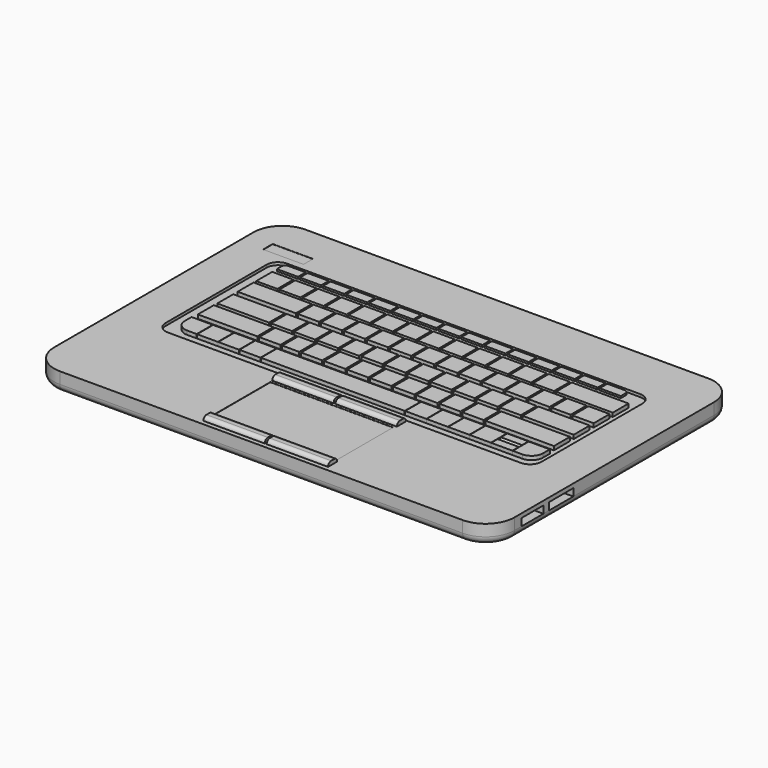
from build123d import *

# Parameters (mm, degrees)
F1_DEPTH  = 12.7
F2_R      = 5.08
F4_DEPTH  = 1.778
F5_W      = 13.7414
F5_H      = 13.2334
F5_W_2    = 13.9954
F5_W_3    = 95.25
F5_H_2    = 13.2237430662
F5_H_3    = 6.6167
F6_DEPTH  = 2.54
F7_SIZE   = 1.27
F8_SIZE   = 1.27
F9_W      = 13.9954
F9_H      = 13.2334
F9_W_2    = 12.7297410883
F9_W_3    = 11.1980646137
F9_W_4    = 13.97
F9_W_5    = 39.3358543515
F9_W_6    = 45.363843441
F9_W_7    = 34.2387035489
F9_W_8    = 33.7878703395
F9_W_9    = 38.5862437279
F9_W_10   = 37.5577136874
F9_H_2    = 13.1128338855
F10_DEPTH = 2.54
F11_W     = 40.64
F11_H     = 7.62
F12_DEPTH = 2.54
F13_R     = 2.53999
F14_R     = 2.53999
F15_R     = 2.53999
F16_W     = 81.28
F16_H     = 46.99
F17_DEPTH = 0.127
F19_DEPTH = 1.27
F18_W     = 13.9954
F18_H     = 6.3754
F20_W     = 26.701785624
F20_H     = 7.8833848238
F21_DEPTH = 0.127
F22_W     = 18.1714147329
F22_H     = 4.8768
F22_W_2   = 19.9380852282
F22_H_2   = 4.8890416828
F23_DEPTH = 12.7


# Not quite as in the source:
# - a fillet or chamfer is up to 0.001 mm smaller than in the source, because OpenCascade refuses the exact size


with BuildPart() as f1:
    # F0 (on Top) → F1 (new body)
    with BuildSketch(Plane.XY):
        with BuildLine():
            Line((133.35, 101.6), (-133.35, 101.6))
            ThreePointArc((-133.35, 101.6), (-146.8203841816, 96.0203841816), (-152.4, 82.55))
            Line((-152.4, 82.55), (-152.4, -82.55))
            ThreePointArc((-152.4, -82.55), (-146.8203841816, -96.0203841816), (-133.35, -101.6))
            Line((-133.35, -101.6), (133.35, -101.6))
            ThreePointArc((133.35, -101.6), (146.8203841816, -96.0203841816), (152.4, -82.55))
            Line((152.4, -82.55), (152.4, 82.55))
            ThreePointArc((152.4, 82.55), (146.8203841816, 96.0203841816), (133.35, 101.6))
        make_face()
    extrude(amount=F1_DEPTH)

    # F2
    f2_edges = [f1.edges().sort_by_distance(p)[0] for p in [
        (0, -101.6, 0),
    ]]
    fillet(f2_edges, radius=F2_R)

    # F3 (on face) → F4 (cut)
    with BuildSketch(Plane.XY.offset(12.7)):
        with BuildLine():
            ThreePointArc((-124.46, -25.1829952943), (-122.2281536726, -30.571148967), (-116.84, -32.8029952943))
            Line((-116.84, -32.8029952943), (116.84, -32.8029952943))
            ThreePointArc((116.84, -32.8029952943), (122.2281536726, -30.571148967), (124.46, -25.1829952943))
            Line((124.46, -25.1829952943), (124.46, 58.3147651076))
            ThreePointArc((124.46, 58.3147651076), (122.2281536726, 63.7029187803), (116.84, 65.9347651076))
            Line((116.84, 65.9347651076), (-116.84, 65.9347651076))
            ThreePointArc((-116.84, 65.9347651076), (-122.2281536726, 63.7029187803), (-124.46, 58.3147651076))
            Line((-124.46, 58.3147651076), (-124.46, -25.1829952943))
        make_face()
    extrude(amount=-F4_DEPTH, mode=Mode.SUBTRACT)

    # F5 (on face) → F6 (join, symmetric)
    with BuildSketch(Plane.XY.offset(10.922)):
        with BuildLine():
            Line((-103.2148086897, -12.7556547022), (-117.2102086897, -12.7556547022))
            Line((-117.2102086897, -12.7556547022), (-117.2102086897, -18.3690547022))
            ThreePointArc((-117.2102086897, -18.3690547022), (-114.9783623623, -23.7572083749), (-109.5902086897, -25.9890547022))
            Line((-109.5902086897, -25.9890547022), (-103.2148086897, -25.9890547022))
            Line((-103.2148086897, -25.9890547022), (-103.2148086897, -12.7556547022))
        make_face()
        with Locations((-96.0901086897, -19.3723547022)):
            Rectangle(F5_W, F5_H)
        with Locations((-82.0947086897, -19.3723547022)):
            Rectangle(F5_W, F5_H)
        with Locations((-67.9723086897, -19.3723547022)):
            Rectangle(F5_W_2, F5_H)
        with Locations((-13.0956086897, -19.3771831691)):
            Rectangle(F5_W_3, F5_H_2)
        with Locations((41.7810913103, -19.3723547022)):
            Rectangle(F5_W_2, F5_H)
        with Locations((56.0304913103, -19.3723547022)):
            Rectangle(F5_W_2, F5_H)
        with Locations((70.2798913103, -19.3723547022)):
            Rectangle(F5_W_2, F5_H)
        Polygon((91.2729913103, -12.7556547022), (77.5315913103, -12.7556547022), (77.5315913103, -25.9890547022), (91.5269913103, -25.9890547022), (91.5269913103, -12.7556547022), align=None)
        with BuildLine():
            Line((120.0257913103, -12.7556547022), (106.0303913103, -12.7556547022))
            Line((106.0303913103, -12.7556547022), (106.0303913103, -25.9890547022))
            Line((106.0303913103, -25.9890547022), (112.4057913103, -25.9890547022))
            ThreePointArc((112.4057913103, -25.9890547022), (117.793944983, -23.7572083749), (120.0257913103, -18.3690547022))
            Line((120.0257913103, -18.3690547022), (120.0257913103, -12.7556547022))
        make_face()
        Polygon((105.7763913103, -19.1183547022), (105.7763913103, -12.6286547022), (91.7809913103, -12.6286547022), (91.7809913103, -19.2453547022), (105.7763913103, -19.2453547022), align=None)
        with Locations((98.7786913103, -22.6807047022)):
            Rectangle(F5_W_2, F5_H_3)
    extrude(amount=F6_DEPTH, both=True)

    # F7
    f7_edges = [f1.edges().sort_by_distance(p)[0] for p in [
        (98.778691, -19.245355, 13.462),
    ]]
    chamfer(f7_edges, length=F7_SIZE)

    # F8
    f8_edges = [f1.edges().sort_by_distance(p)[0] for p in [
        (98.778691, -19.372355, 13.462),
    ]]
    chamfer(f8_edges, length=F8_SIZE)

    # F9 (on face) → F10 (join)
    with BuildSketch(Plane.XY.offset(10.922)):
        with Locations((-69.4690281525, 30.8539665655)):
            Rectangle(F9_W, F9_H)
        with Locations((-54.2036281525, 30.8539665655)):
            Rectangle(F9_W, F9_H)
        Polygon((-31.9405281525, 24.2372665655), (-31.9405281525, 37.4706665655), (-34.4356895394, 37.4706665655), (-45.9359281525, 37.4706665655), (-45.9359281525, 24.2372665655), align=None)
        Polygon((-16.6751281525, 37.4187609684), (-30.6705281525, 37.4814295383), (-30.6705281525, 24.2480295383), (-16.6751281525, 24.2480295383), align=None)
        with Locations((22.1233718475, 30.8539665655)):
            Rectangle(F9_W, F9_H)
        with Locations((37.3887718475, 30.8539665655)):
            Rectangle(F9_W, F9_H)
        with Locations((6.8579718475, 30.8539665655)):
            Rectangle(F9_W, F9_H)
        with Locations((-8.4074281525, 30.8539665655)):
            Rectangle(F9_W, F9_H)
        with Locations((52.6541718475, 30.8539665655)):
            Rectangle(F9_W, F9_H)
        with Locations((67.9195718475, 30.8539665655)):
            Rectangle(F9_W, F9_H)
        with Locations((97.8175423916, 30.8539665655)):
            Rectangle(F9_W_2, F9_H)
        with Locations((83.1849718475, 30.8539665655)):
            Rectangle(F9_W, F9_H)
        with Locations((-41.1575174346, -1.8301518617)):
            Rectangle(F9_W, F9_H)
        with Locations((-68.8909820483, -1.8301518617)):
            Rectangle(F9_W, F9_H)
        with Locations((65.7002825654, -1.9120993343)):
            Rectangle(F9_W, F9_H)
        with Locations((19.9040825654, -1.9120993343)):
            Rectangle(F9_W, F9_H)
        with Locations((4.6386825654, -1.9120993343)):
            Rectangle(F9_W, F9_H)
        with Locations((-55.0242497415, -1.8301518617)):
            Rectangle(F9_W_3, F9_H)
        with Locations((50.4348825654, -1.9120993343)):
            Rectangle(F9_W, F9_H)
        with Locations((-10.6267174346, -1.9120993343)):
            Rectangle(F9_W, F9_H)
        with Locations((35.1694825654, -1.9120993343)):
            Rectangle(F9_W, F9_H)
        with Locations((-25.8921174346, -1.8301518617)):
            Rectangle(F9_W, F9_H)
        with Locations((62.0888653013, 14.3678454001)):
            Rectangle(F9_W, F9_H)
        with Locations((-43.2857683315, 14.0165393491)):
            Rectangle(F9_W, F9_H)
        with Locations((-73.8165683315, 14.0165393491)):
            Rectangle(F9_W, F9_H)
        with Locations((-58.5511683315, 14.0165393491)):
            Rectangle(F9_W, F9_H)
        with Locations((31.5580653013, 14.3678454001)):
            Rectangle(F9_W, F9_H)
        with Locations((16.2926653013, 14.3678454001)):
            Rectangle(F9_W, F9_H)
        with Locations((46.8234653013, 14.3678454001)):
            Rectangle(F9_W, F9_H)
        with Locations((1.0272653013, 14.3678454001)):
            Rectangle(F9_W, F9_H)
        with Locations((77.3542653013, 14.3678454001)):
            Rectangle(F9_W, F9_H)
        with Locations((-14.2381346987, 14.3678454001)):
            Rectangle(F9_W, F9_H)
        Polygon((-22.5058346987, 20.6349561019), (-35.0180683315, 20.6332393491), (-35.0180683315, 7.3998393491), (-22.5058346987, 7.3998393491), align=None)
        with Locations((-78.7226834506, 46.1651931025)):
            Rectangle(F9_W, F9_H)
        with Locations((12.8697165494, 46.1651931025)):
            Rectangle(F9_W, F9_H)
        with Locations((-17.6610834506, 46.1651931025)):
            Rectangle(F9_W, F9_H)
        Polygon((-41.1941834506, 39.5484931025), (-41.1941834506, 52.7818931025), (-48.679478426, 52.7818931025), (-51.2247426917, 52.7818931025), (-55.1895834506, 52.7818931025), (-55.1895834506, 39.6280735731), align=None)
        with Locations((-109.2534834506, 46.1651931025)):
            Rectangle(F9_W, F9_H)
        with Locations((28.1351165494, 46.1651931025)):
            Rectangle(F9_W, F9_H)
        with Locations((73.9059165494, 46.1651931025)):
            Rectangle(F9_W, F9_H)
        with Locations((-63.4572834506, 46.1651931025)):
            Rectangle(F9_W, F9_H)
        Polygon((-6.4493968805, 52.7818931025), (-9.3933834506, 52.7818931025), (-9.3933834506, 39.5484931025), (4.6020165494, 39.5484931025), (4.6020165494, 52.7818931025), (-3.9041326148, 52.7818931025), align=None)
        with Locations((-93.9880834506, 46.1651931025)):
            Rectangle(F9_W, F9_H)
        with Locations((-32.9264834506, 46.1651931025)):
            Rectangle(F9_W, F9_H)
        with Locations((43.4005165494, 46.1651931025)):
            Rectangle(F9_W, F9_H)
        with Locations((58.6532165494, 46.1651931025)):
            Rectangle(F9_W_4, F9_H)
        with Locations((-96.8266092241, -1.8301518617)):
            Rectangle(F9_W_5, F9_H)
        with Locations((96.6499042859, -1.9120993343)):
            Rectangle(F9_W_6, F9_H)
        with Locations((-99.203620106, 14.0165393491)):
            Rectangle(F9_W_7, F9_H)
        with Locations((102.5159004711, 14.3678454001)):
            Rectangle(F9_W_8, F9_H)
        with Locations((-97.0298500165, 30.8539665655)):
            Rectangle(F9_W_9, F9_H)
        with Locations((100.9524733932, 46.2254761597)):
            Rectangle(F9_W_10, F9_H_2)
        with Locations((112.4501129357, 30.8539665655)):
            Rectangle(F9_W, F9_H)
    extrude(amount=F10_DEPTH)

    # F11 (on face) → F12 (join)
    with BuildSketch(Plane.XY.offset(12.7)):
        with Locations((21.1591962329, -37.3785455251)):
            Rectangle(F11_W, F11_H)
        with Locations((-20.7508037671, -37.3785455251)):
            Rectangle(F11_W, F11_H)
        with Locations((21.5003191698, -94.7764143348)):
            Rectangle(F11_W, F11_H)
        with Locations((-20.4096808302, -94.7764143348)):
            Rectangle(F11_W, F11_H)
    extrude(amount=F12_DEPTH)

    # F13 (radius 2.54 in the source; OpenCascade refuses exactly that, so slightly less here)
    f13_edges = [f1.edges().sort_by_distance(p)[0] for p in [
        (21.159196, -41.188546, 15.24),
        (21.159196, -33.568546, 15.24),
    ]]
    fillet(f13_edges, radius=F13_R)

    # F14 (radius 2.54 in the source; OpenCascade refuses exactly that, so slightly less here)
    f14_edges = [f1.edges().sort_by_distance(p)[0] for p in [
        (-20.750804, -41.188546, 15.24),
        (-20.750804, -33.568546, 15.24),
        (-20.409681, -90.966414, 15.24),
        (21.500319, -90.966414, 15.24),
    ]]
    fillet(f14_edges, radius=F14_R)

    # F15 (radius 2.54 in the source; OpenCascade refuses exactly that, so slightly less here)
    f15_edges = [f1.edges().sort_by_distance(p)[0] for p in [
        (-20.409681, -98.586414, 15.24),
        (21.500319, -98.586414, 15.24),
    ]]
    fillet(f15_edges, radius=F15_R)

    # F16 (on face) → F17 (cut)
    with BuildSketch(Plane.XY.offset(12.7)):
        with Locations((-0.1672953367, -66.5201838687)):
            Rectangle(F16_W, F16_H)
    extrude(amount=-F17_DEPTH, mode=Mode.SUBTRACT)

    # F20 (on face) → F21 (cut)
    with BuildSketch(Plane.XY.offset(12.7)):
        with Locations((-123.120021075, 74.5107010007)):
            Rectangle(F20_W, F20_H)
    extrude(amount=-F21_DEPTH, mode=Mode.SUBTRACT)

    # F22 (on face) → F23 (cut)
    with BuildSketch(Plane.YZ.offset(152.4)):
        with Locations((-67.6380544901, 7.5184)):
            Rectangle(F22_W, F22_H)
        with Locations((-43.7880698591, 7.5245208414)):
            Rectangle(F22_W_2, F22_H_2)
    extrude(amount=-F23_DEPTH, mode=Mode.SUBTRACT)


with BuildPart() as f19:
    # F18 (on face) → F19 (new body)
    with BuildSketch(Plane.XY.offset(12.7)):
        with BuildLine():
            Line((-101.7563656684, 62.3987905988), (-113.2117656684, 62.3987905988))
            ThreePointArc((-113.2117656684, 62.3987905988), (-115.0078168926, 61.654841823), (-115.7517656684, 59.8587905988))
            Line((-115.7517656684, 59.8587905988), (-115.7517656684, 56.010723114))
            Line((-115.7517656684, 56.010723114), (-101.7563656684, 56.010723114))
            Line((-101.7563656684, 56.010723114), (-101.7563656684, 62.3987905988))
        make_face()
    extrude(amount=F19_DEPTH)


with BuildPart() as f19b:
    # F18 (on face) → F19, piece 2 (new body)
    with BuildSketch(Plane.XY.offset(12.7)):
        with Locations((-93.4886656684, 59.2110905988)):
            Rectangle(F18_W, F18_H)
    extrude(amount=F19_DEPTH)


with BuildPart() as f19c:
    # F18 (on face) → F19, piece 3 (new body)
    with BuildSketch(Plane.XY.offset(12.7)):
        with Locations((-78.2232656684, 59.2110905988)):
            Rectangle(F18_W, F18_H)
    extrude(amount=F19_DEPTH)


with BuildPart() as f19d:
    # F18 (on face) → F19, piece 4 (new body)
    with BuildSketch(Plane.XY.offset(12.7)):
        with Locations((-47.6924656684, 59.2110905988)):
            Rectangle(F18_W, F18_H)
    extrude(amount=F19_DEPTH)


with BuildPart() as f19e:
    # F18 (on face) → F19, piece 5 (new body)
    with BuildSketch(Plane.XY.offset(12.7)):
        with Locations((-62.9578656684, 59.2110905988)):
            Rectangle(F18_W, F18_H)
    extrude(amount=F19_DEPTH)


with BuildPart() as f19f:
    # F18 (on face) → F19, piece 6 (new body)
    with BuildSketch(Plane.XY.offset(12.7)):
        with Locations((-17.1616656684, 59.2110905988)):
            Rectangle(F18_W, F18_H)
    extrude(amount=F19_DEPTH)


with BuildPart() as f19g:
    # F18 (on face) → F19, piece 7 (new body)
    with BuildSketch(Plane.XY.offset(12.7)):
        with Locations((-32.4270656684, 59.2110905988)):
            Rectangle(F18_W, F18_H)
    extrude(amount=F19_DEPTH)


with BuildPart() as f19h:
    # F18 (on face) → F19, piece 8 (new body)
    with BuildSketch(Plane.XY.offset(12.7)):
        with Locations((13.3691343316, 59.2110905988)):
            Rectangle(F18_W, F18_H)
    extrude(amount=F19_DEPTH)


with BuildPart() as f19i:
    # F18 (on face) → F19, piece 9 (new body)
    with BuildSketch(Plane.XY.offset(12.7)):
        with Locations((-1.8962656684, 59.2110905988)):
            Rectangle(F18_W, F18_H)
    extrude(amount=F19_DEPTH)


with BuildPart() as f19j:
    # F18 (on face) → F19, piece 10 (new body)
    with BuildSketch(Plane.XY.offset(12.7)):
        with Locations((43.8999343316, 59.2110905988)):
            Rectangle(F18_W, F18_H)
    extrude(amount=F19_DEPTH)


with BuildPart() as f19k:
    # F18 (on face) → F19, piece 11 (new body)
    with BuildSketch(Plane.XY.offset(12.7)):
        with Locations((28.6345343316, 59.2110905988)):
            Rectangle(F18_W, F18_H)
    extrude(amount=F19_DEPTH)


with BuildPart() as f19l:
    # F18 (on face) → F19, piece 12 (new body)
    with BuildSketch(Plane.XY.offset(12.7)):
        with Locations((74.4307343316, 59.2110905988)):
            Rectangle(F18_W, F18_H)
    extrude(amount=F19_DEPTH)


with BuildPart() as f19m:
    # F18 (on face) → F19, piece 13 (new body)
    with BuildSketch(Plane.XY.offset(12.7)):
        with Locations((59.1653343316, 59.2110905988)):
            Rectangle(F18_W, F18_H)
    extrude(amount=F19_DEPTH)


with BuildPart() as f19n:
    # F18 (on face) → F19, piece 14 (new body)
    with BuildSketch(Plane.XY.offset(12.7)):
        with BuildLine():
            Line((109.4192343316, 62.3987905988), (97.9638343316, 62.3987905988))
            Line((97.9638343316, 62.3987905988), (97.9638343316, 56.0233905988))
            Line((97.9638343316, 56.0233905988), (111.9592343316, 56.0233905988))
            Line((111.9592343316, 56.0233905988), (111.9592343316, 59.8587905988))
            ThreePointArc((111.9592343316, 59.8587905988), (111.2152855558, 61.654841823), (109.4192343316, 62.3987905988))
        make_face()
    extrude(amount=F19_DEPTH)


with BuildPart() as f19o:
    # F18 (on face) → F19, piece 15 (new body)
    with BuildSketch(Plane.XY.offset(12.7)):
        with Locations((89.6961343316, 59.2110905988)):
            Rectangle(F18_W, F18_H)
    extrude(amount=F19_DEPTH)


solid = Compound([f1.part, f19.part, f19b.part, f19c.part, f19d.part, f19e.part, f19f.part, f19g.part, f19h.part, f19i.part, f19j.part, f19k.part, f19l.part, f19m.part, f19n.part, f19o.part])
